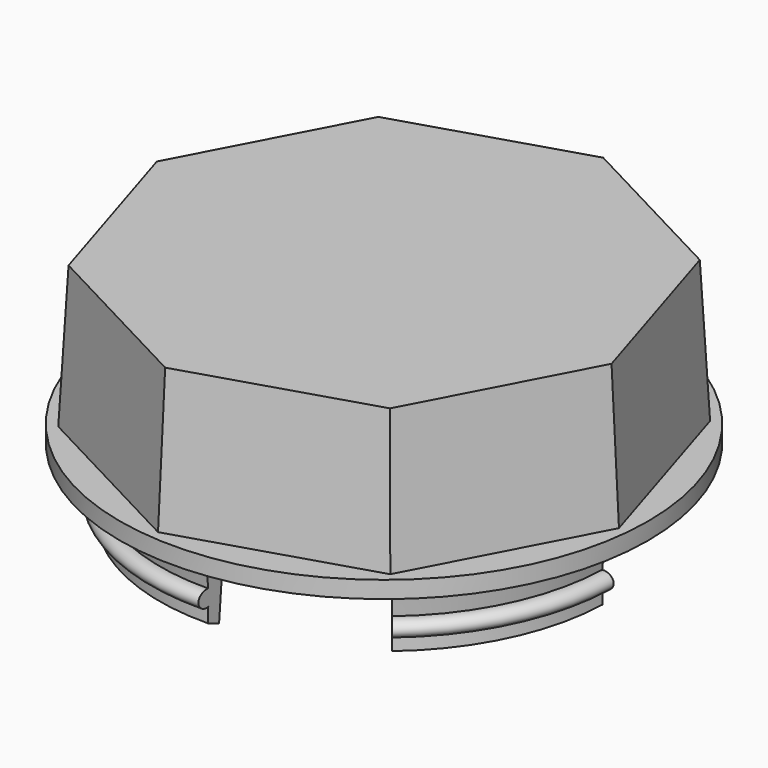
from build123d import *

# Parameters (mm, degrees)
F1_DEPTH  = 19.6
F1_TAPER  = 3
F6_R      = 29.5588051004
F7_DEPTH  = 17
F10_START = -5
F10_DEPTH = 20
F13_DEPTH = 10


# Not quite as in the source:
# - the program builds the solid bodies; features that only make, move or delete a surface that nothing else refers to are left out


with BuildPart() as f1:
    # F0 (on Top) → F1 (new body)
    with BuildSketch(Plane.XY):
        Polygon((6.846458452, 3.2292531715), (14.8228506263, -22.4859673376), (38.6464184239, -35.0292131433), (64.3616389329, -27.052820969), (76.9048847387, -3.2292531715), (68.9284925643, 22.4859673376), (45.1049247668, 35.0292131433), (19.3897042578, 27.052820969), align=None)
    extrude(amount=F1_DEPTH, taper=F1_TAPER)

    # F6 (on Top) → F7 (cut)
    with BuildSketch(Plane.XY):
        with Locations((41.8770387769, 0)):
            Circle(F6_R)
    extrude(amount=F7_DEPTH, mode=Mode.SUBTRACT)


with BuildPart() as f5:
    # F4 (on Front) → F5 (revolve)
    with BuildSketch(Plane.XZ):
        with BuildLine():
            Line((12.6976181568, -12.3096757326), (13.6948058819, 0))
            Line((13.6948058819, 0), (10.6566109201, 0))
            Line((10.6566109201, 0), (5.3524481356, 0))
            Line((5.3524481356, 0), (5.3524481356, -2.35))
            Line((5.3524481356, -2.35), (10.3524481356, -2.35))
            Line((10.3524481356, -2.35), (10.9037844754, -7.3195098592))
            add(Edge.make_bspline(
                [(10.9037844754, -7.3195098592), (9.9054742604, -7.188339252), (8.526802396, -8.5542281967), (10.0830420852, -9.7186826169), (10.9037844754, -9.5387469869)],
                knots=[0, 0, 0, 0, 0.5064173363, 1, 1, 1, 1], degree=3))
            Line((10.9037844754, -9.5387469869), (10.8524481356, -11.5380880234))
            Line((10.8524481356, -11.5380880234), (12.6976181568, -12.3096757326))
        make_face()
    revolve(axis=Axis((41.8524481356, 0, -10.1716983277), (0, 0, -1)))


with BuildPart() as f10:
    # F9 (on Top) → F10 (new body)
    with BuildSketch(Plane.XY.offset(F10_START)):
        Polygon((42.6140986383, -43.1583486497), (69.8464736342, -34.131936729), (60.4310854986, -22.0097155725), (42.8283442474, -28.884228869), align=None)
        Polygon((42.8283442474, -28.884228869), (60.4310854986, -22.0097155725), (43.3466422396, -0.013660122), (43.260671187, -0.0804342567), align=None)
        Polygon((43.260671187, -0.0804342567), (43.3466422396, -0.013660122), (43.3372866763, -0.0016149246), (43.2618701985, -0.0005500774), align=None)
        Polygon((43.3372866763, -0.0016149246), (43.3466422396, -0.013660122), (43.3617063937, -0.0019597202), align=None)
        Polygon((43.2618701985, -0.0005500774), (43.3372866763, -0.0016149246), (43.2632842698, 0.093662458), align=None)
        Polygon((19.4793593917, -18.5514948023), (43.260671187, -0.0804342567), (43.2618701985, -0.0005500774), (43.2229116559, 0), (12.5911462439, 0.4803054209), align=None)
        Polygon((9.1356113553, -26.585534215), (19.4793593917, -18.5514948023), (12.5911462439, 0.4803054209), (0, 0.6777343224), align=None)
    extrude(amount=-F10_DEPTH)


with BuildPart() as f10b:
    # F9 (on Top) → F10, piece 2 (new body)
    with BuildSketch(Plane.XY.offset(F10_START)):
        Polygon((24.825832521, 23.8317032525), (43.2632842698, 0.093662458), (43.6881296354, 28.3989969936), align=None)
        Polygon((16.3248591125, 34.7766242921), (24.825832521, 23.8317032525), (43.6881296354, 28.3989969936), (43.9111739397, 43.2593300939), align=None)
    extrude(amount=-F10_DEPTH)


with BuildPart() as f10c:
    # F9 (on Top) → F10, piece 3 (new body)
    with BuildSketch(Plane.XY.offset(F10_START)):
        Polygon((65.2221173543, 16.9771278037), (43.3617063937, -0.0019597202), (71.1709585301, -0.3946140477), align=None)
        Polygon((79.0283353161, 27.7004844491), (65.2221173543, 16.9771278037), (71.1709585301, -0.3946140477), (86.5694135427, -0.6120334147), align=None)
    extrude(amount=-F10_DEPTH)


with BuildPart() as f5_1:
    add(f5.part)

    # F11: cut F10, F10c, F10b
    add(f10.part, mode=Mode.SUBTRACT)
    add(f10c.part, mode=Mode.SUBTRACT)
    add(f10b.part, mode=Mode.SUBTRACT)


with BuildPart() as f13:
    # F12 (on Top) → F13 (new body)
    with BuildSketch(Plane.XY):
        Polygon((81.2726734822, 21.7885523797), (76.6011070263, 26.0260878816), (43.354075402, 0), align=None)
    extrude(amount=-F13_DEPTH)


with BuildPart() as f13b:
    # F12 (on Top) → F13, piece 2 (new body)
    with BuildSketch(Plane.XY):
        Polygon((85.3246003462, 4.6040632222), (43.354075402, 0), (87.0625718818, -1.4589142), align=None)
    extrude(amount=-F13_DEPTH)


with BuildPart() as f13c:
    # F12 (on Top) → F13, piece 3 (new body)
    with BuildSketch(Plane.XY):
        Polygon((74.1051476533, -39.282963935), (43.354075402, 0), (69.7669919231, -45.9663748299), align=None)
    extrude(amount=-F13_DEPTH)


with BuildPart() as f13d:
    # F12 (on Top) → F13, piece 4 (new body)
    with BuildSketch(Plane.XY):
        Polygon((48.7939971237, -49.5901900761), (43.354075402, 0), (41.5855238111, -52.9851111108), align=None)
    extrude(amount=-F13_DEPTH)


with BuildPart() as f13e:
    # F12 (on Top) → F13, piece 5 (new body)
    with BuildSketch(Plane.XY):
        Polygon((5.9819950958, -29.2552146417), (43.354075402, 0), (1.6118744296, -23.9856476341), align=None)
    extrude(amount=-F13_DEPTH)


with BuildPart() as f13f:
    # F12 (on Top) → F13, piece 6 (new body)
    with BuildSketch(Plane.XY):
        Polygon((-3.8238455154, -5.1753017358), (43.354075402, 0), (-4.7618607516, 1.6060269319), align=None)
    extrude(amount=-F13_DEPTH)


with BuildPart() as f13g:
    # F12 (on Top) → F13, piece 7 (new body)
    with BuildSketch(Plane.XY):
        Polygon((14.7173287406, 36.5820182504), (43.354075402, 0), (20.0315345828, 40.5881967797), align=None)
    extrude(amount=-F13_DEPTH)


with BuildPart() as f13h:
    # F12 (on Top) → F13, piece 8 (new body)
    with BuildSketch(Plane.XY):
        Polygon((38.2881817991, 46.1805591199), (43.354075402, 0), (44.9157021402, 46.7857237843), align=None)
    extrude(amount=-F13_DEPTH)


with BuildPart() as f13g_1:
    # F14: moved
    add(f13g.part.moved(Location((0, 0, -2.35))))


with BuildPart() as f13f_1:
    # F14: moved
    add(f13f.part.moved(Location((0, 0, -2.35))))


with BuildPart() as f13e_1:
    # F14: moved
    add(f13e.part.moved(Location((0, 0, -2.35))))


with BuildPart() as f13d_1:
    # F14: moved
    add(f13d.part.moved(Location((0, 0, -2.35))))


with BuildPart() as f13c_1:
    # F14: moved
    add(f13c.part.moved(Location((0, 0, -2.35))))


with BuildPart() as f13b_1:
    # F14: moved
    add(f13b.part.moved(Location((0, 0, -2.35))))


with BuildPart() as f13_1:
    # F14: moved
    add(f13.part.moved(Location((0, 0, -2.35))))


with BuildPart() as f13h_1:
    # F14: moved
    add(f13h.part.moved(Location((0, 0, -2.35))))


with BuildPart() as f5_2:
    add(f5_1.part)

    # F15: cut F13g, F13f, F13e, F13d, F13c, F13b, F13, F13h
    add(f13g_1.part, mode=Mode.SUBTRACT)
    add(f13f_1.part, mode=Mode.SUBTRACT)
    add(f13e_1.part, mode=Mode.SUBTRACT)
    add(f13d_1.part, mode=Mode.SUBTRACT)
    add(f13c_1.part, mode=Mode.SUBTRACT)
    add(f13b_1.part, mode=Mode.SUBTRACT)
    add(f13_1.part, mode=Mode.SUBTRACT)
    add(f13h_1.part, mode=Mode.SUBTRACT)


solid = Compound([f1.part, f5_2.part])
